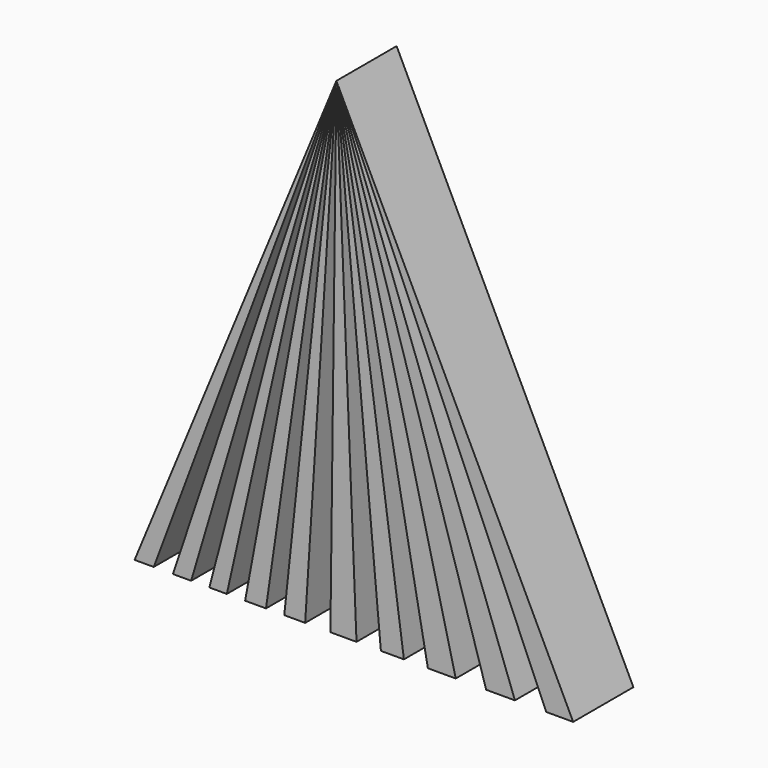
from build123d import *

# Parameters (mm, degrees)
F1_DEPTH = 25.4


# Not quite as in the source:
# - a feature names something its author has since deleted; it is built from what else it names


with BuildPart() as f1:
    # F0 (on Front) → F1 (new body)
    with BuildSketch(Plane.XZ):
        Polygon((-22.78999798, 164.4750535488), (-90.8892974257, 0), (-84.4279974699, 0), align=None)
    extrude(amount=F1_DEPTH)


with BuildPart() as f1b:
    # F0 (on Front) → F1, piece 2 (new body)
    with BuildSketch(Plane.XZ):
        Polygon((-71.8118920922, 0), (-22.78999798, 164.4750535488), (-77.9664888978, 0), align=None)
    extrude(amount=F1_DEPTH)


with BuildPart() as f1c:
    # F0 (on Front) → F1, piece 3 (new body)
    with BuildSketch(Plane.XZ):
        Polygon((-59.7685277462, 0), (-22.78999798, 164.4750535488), (-65.6433403492, 0), align=None)
    extrude(amount=F1_DEPTH)


with BuildPart() as f1d:
    # F0 (on Front) → F1, piece 4 (new body)
    with BuildSketch(Plane.XZ):
        Polygon((-46.5501956642, 0), (-22.78999798, 164.4750535488), (-53.5999722779, 0), align=None)
    extrude(amount=F1_DEPTH)


with BuildPart() as f1e:
    # F0 (on Front) → F1, piece 5 (new body)
    with BuildSketch(Plane.XZ):
        Polygon((-33.3318635821, 0), (-22.78999798, 164.4750535488), (-40.3816401958, 0), align=None)
    extrude(amount=F1_DEPTH)


with BuildPart() as f1f:
    # F0 (on Front) → F1, piece 6 (new body)
    with BuildSketch(Plane.XZ):
        Polygon((-16.0011649132, 0), (-22.78999798, 164.4750535488), (-24.813387543, 0), align=None)
    extrude(amount=F1_DEPTH)


with BuildPart() as f1g:
    # F0 (on Front) → F1, piece 7 (new body)
    with BuildSketch(Plane.XZ):
        Polygon((0, 0), (-22.78999798, 164.4750535488), (-7.7764266171, 0), align=None)
    extrude(amount=F1_DEPTH)


with BuildPart() as f1h:
    # F0 (on Front) → F1, piece 8 (new body)
    with BuildSketch(Plane.XZ):
        Polygon((17.4852721393, 0), (-22.78999798, 164.4750535488), (8.0855702981, 0), align=None)
    extrude(amount=F1_DEPTH)


with BuildPart() as f1i:
    # F0 (on Front) → F1, piece 9 (new body)
    with BuildSketch(Plane.XZ):
        Polygon((37.4596379697, 0), (-22.78999798, 164.4750535488), (27.7661941946, 0), align=None)
    extrude(amount=F1_DEPTH)


with BuildPart() as f1j:
    # F0 (on Front) → F1, piece 10 (new body)
    with BuildSketch(Plane.XZ):
        Polygon((57.1233406663, 0), (-22.78999798, 164.4750535488), (48.0343028903, 0), align=None)
    extrude(amount=F1_DEPTH)


solid = Compound([f1.part, f1b.part, f1c.part, f1d.part, f1e.part, f1f.part, f1g.part, f1h.part, f1i.part, f1j.part])
